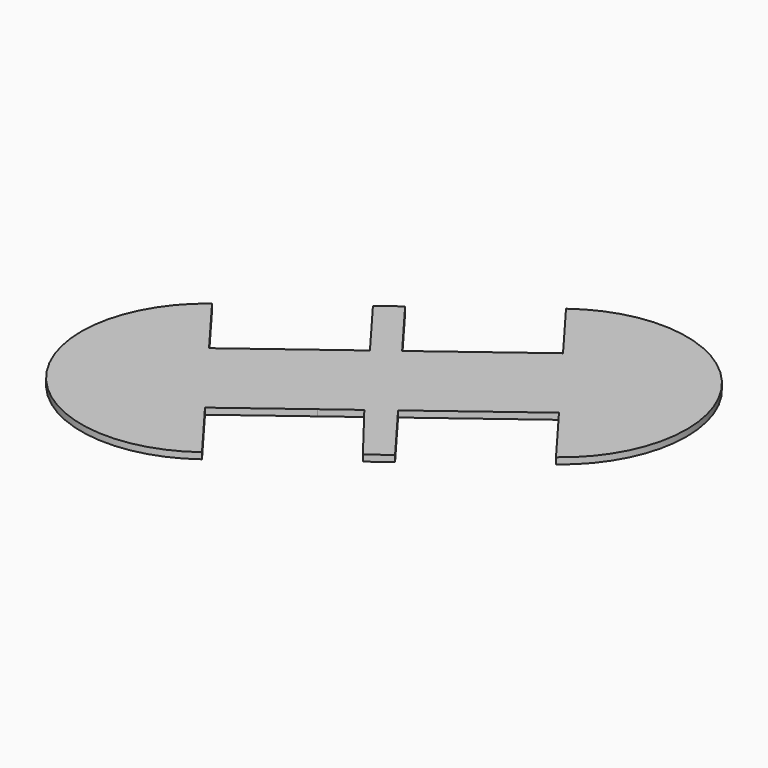
from build123d import *

# Parameters (mm, degrees)
F1_DEPTH = 3.175
F3_DEPTH = 50.8
F4_R     = 6.35
F5_DEPTH = 50.8


# Not quite as in the source:
# - a length typed as a fraction of an inch, garbled in the dataset ("3 / 203.2 mm" for 3/8 in), is restored


with BuildPart() as f1:
    # F0 (on Top) → F1 (new body)
    with BuildSketch(Plane.XY):
        with BuildLine():
            Line((53.34, -21.8826867197), (76.2, -52.3626867197))
            ThreePointArc((76.2, -52.3626867197), (88.9, 36.5373132803), (0, 49.2373132803))
            Line((0, 49.2373132803), (22.86, 18.7573132803))
            Line((22.86, 18.7573132803), (-27.94, -19.3426867197))
            Line((-27.94, -19.3426867197), (-50.8, 11.1373132803))
            Line((-50.8, 11.1373132803), (-60.96, 3.5173132803))
            Line((-60.96, 3.5173132803), (-38.1, -26.9626867197))
            Line((-38.1, -26.9626867197), (-88.9, -65.0626867197))
            Line((-88.9, -65.0626867197), (-111.76, -34.5826867197))
            ThreePointArc((-111.76, -34.5826867197), (-124.46, -123.4826867197), (-35.56, -136.1826867197))
            Line((-35.56, -136.1826867197), (-58.42, -105.7026867197))
            Line((-58.42, -105.7026867197), (-22.9741035603, -79.11826439))
            Line((-22.9741035603, -79.11826439), (-8.1111921991, -67.971080869))
            Line((-8.1111921991, -67.971080869), (15.24, -98.0826867197))
            Line((15.24, -98.0826867197), (25.4, -90.4626867197))
            Line((25.4, -90.4626867197), (2.54, -59.9826867197))
            Line((2.54, -59.9826867197), (53.34, -21.8826867197))
        make_face()
    extrude(amount=F1_DEPTH)

    # F2 (on face) → F3 (cut)
    with BuildSketch(Plane(origin=(29.7060896255, -39.6081195006, 0), x_dir=(0.8, 0.6, 0), z_dir=(0.6, -0.8, 0))):
        with BuildLine():
            ThreePointArc((-78.7146071563, -9.525), (-83.2047352168, -20.3651280605), (-72.3646071563, -15.875))
            ThreePointArc((-72.3646071563, -15.875), (-74.2244790957, -11.3848719395), (-78.7146071563, -9.525))
        make_face()
    extrude(amount=-F3_DEPTH, mode=Mode.SUBTRACT)

    # F4 (on face) → F5 (cut)
    with BuildSketch(Plane(origin=(-0.7739103745, 1.0318804994, 0), x_dir=(-0.8, -0.6, 0), z_dir=(-0.6, 0.8, 0))):
        with Locations((2.2076120318, -15.875)):
            Circle(F4_R)
    extrude(amount=-F5_DEPTH, mode=Mode.SUBTRACT)


solid = f1.part
